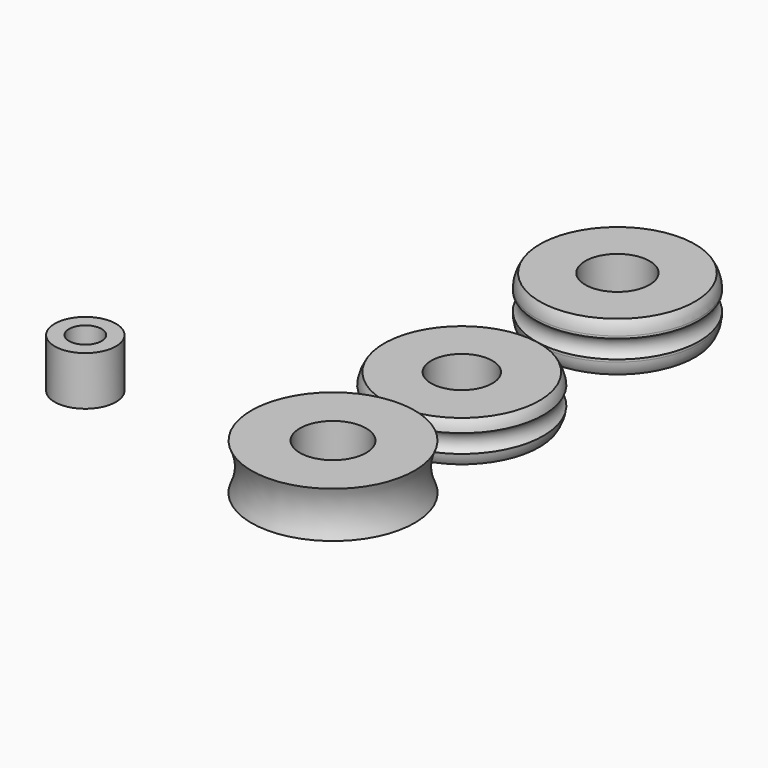
from build123d import *

# Parameters (mm, degrees)
F0_R           = 3
F0_R_2         = 1.6
F1_DEPTH       = 4
F0_R_3         = 8
F2_DEPTH       = 0.8
F3_R           = 3
F4_DEPTH       = 25
F4_DEPTH_BACK  = 25
F11_DEPTH      = 0.8
F12_R          = 3.15
F13_DEPTH      = 25
F13_DEPTH_BACK = 25
F14_R          = 8
F14_R_2        = 3.25
F15_DEPTH      = 4.5


with BuildPart() as f1:
    # F0 (on Top) → F1 (new body)
    with BuildSketch(Plane.XY):
        with Locations((-25.3434665501, 1.3662634883)):
            Circle(F0_R)
        with Locations((-25.3434665501, 1.3662634883)):
            Circle(F0_R_2, mode=Mode.SUBTRACT)
    extrude(amount=F1_DEPTH)

    # F11 (add): a face of the model
    f11_faces = [f1.faces().sort_by_distance(p)[0] for p in [
        (-28.2586137364, 1.3662634883, 4),
    ]]
    extrude(f11_faces, amount=F11_DEPTH)


with BuildPart() as f1b:
    # F0 (on Top) → F1, piece 2 (new body)
    with BuildSketch(Plane.XY):
        with Locations((0, 15.7561581582)):
            Circle(F0_R_3)
    extrude(amount=F1_DEPTH)


with BuildPart() as f1c:
    # F0 (on Top) → F1, piece 3 (new body)
    with BuildSketch(Plane.XY):
        with Locations((0, 34.8054356873)):
            Circle(F0_R_3)
    extrude(amount=F1_DEPTH)

    # F2 (add): a face of the model
    f2_faces = [f1c.faces().sort_by_distance(p)[0] for p in [
        (0, 34.8054356873, 4),
    ]]
    extrude(f2_faces, amount=F2_DEPTH)


with BuildPart() as f4_tool:
    # F3 (on face) → F4 (new body, two sides)
    with BuildSketch(Plane.XY.offset(4)) as f4_sk:
        with Locations((0, 15.7561581582)):
            Circle(F3_R)
        with Locations((0, 34.8054356873)):
            Circle(F3_R)
    extrude(amount=-F4_DEPTH)
    extrude(f4_sk.sketch, amount=F4_DEPTH_BACK)


with BuildPart() as f1b_1:
    add(f1b.part)

    # F4: cut by f4_tool
    add(f4_tool.part, mode=Mode.SUBTRACT)

    # F6 (on Right) → F7 (revolve, cut)
    with BuildSketch(Plane.YZ):
        with BuildLine():
            ThreePointArc((8.1561581582, 0), (7.8928465089, 0.5298800346), (7.7561581582, 1.105572809))
            ThreePointArc((7.7561581582, 1.105572809), (8.1561581582, 2), (7.7561581582, 2.894427191))
            ThreePointArc((7.7561581582, 2.894427191), (7.8928465089, 3.4701199654), (8.1561581582, 4))
            Line((8.1561581582, 4), (7.7561581582, 4))
            Line((7.7561581582, 4), (1.3885094086, 4))
            Line((1.3885094086, 4), (1.3885094086, 0))
            Line((1.3885094086, 0), (8.1561581582, 0))
        make_face()
    revolve(axis=Axis((0, 15.7561581582, 3), (0, 0, -1)), mode=Mode.SUBTRACT)


with BuildPart() as f1c_1:
    add(f1c.part)

    # F4: cut by f4_tool
    add(f4_tool.part, mode=Mode.SUBTRACT)

    # F9 (on Right) → F10 (revolve, cut)
    with BuildSketch(Plane.YZ):
        with BuildLine():
            ThreePointArc((27.2054356873, 0), (26.8900265118, 0.7221245395), (26.8054356873, 1.505572809))
            ThreePointArc((26.8054356873, 1.505572809), (27.2054356873, 2.4), (26.8054356873, 3.294427191))
            ThreePointArc((26.8054356873, 3.294427191), (26.8900265118, 4.0778754605), (27.2054356873, 4.8))
            ThreePointArc((27.2054356873, 4.8), (9.199474241, 2.4), (27.2054356873, 0))
        make_face()
    revolve(axis=Axis((0, 34.8054356873, 3.6), (0, 0, -1)), mode=Mode.SUBTRACT)

    # F12 (on face) → F13 (cut, two sides)
    with BuildSketch(Plane.XY.offset(4.8)) as f13_sk:
        with Locations((0, 34.8054356873)):
            Circle(F12_R)
        with Locations((0, 15.7561581582)):
            Circle(F12_R)
    extrude(amount=-F13_DEPTH, mode=Mode.SUBTRACT)
    extrude(f13_sk.sketch, amount=F13_DEPTH_BACK, mode=Mode.SUBTRACT)


with BuildPart() as f15:
    # F14 (on Top) → F15 (new body)
    with BuildSketch(Plane.XY):
        Circle(F14_R)
        Circle(F14_R_2, mode=Mode.SUBTRACT)
    extrude(amount=F15_DEPTH)

    # F16 (on Right) → F17 (revolve, cut)
    with BuildSketch(Plane.YZ):
        with BuildLine():
            ThreePointArc((-8, 4.5229381791), (-17.8737479846, 2.2614690895), (-8, 0))
            ThreePointArc((-8, 0), (-7.5, 2.2614690895), (-8, 4.5229381791))
        make_face()
    revolve(axis=Axis((0, 0, 2.25), (0, 0, -1)), mode=Mode.SUBTRACT)


solid = Compound([f1.part, f1b_1.part, f1c_1.part, f15.part])
